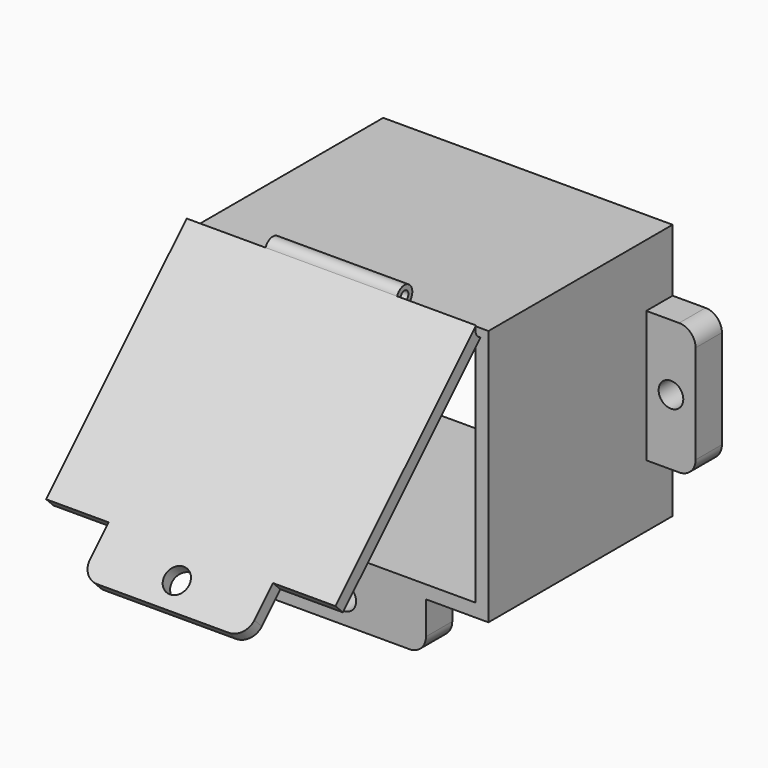
from build123d import *

# Parameters (mm, degrees)
F0_W           = 80
F0_H           = 70
F1_DEPTH       = 70
F0_W_2         = 15
F0_H_2         = 40
F0_R           = 3.75
F2_DEPTH       = 10
F3_R           = 5
F6_W           = 50
F6_H           = 15
F6_R           = 3.75
F7_DEPTH       = 10
F8_R           = 5
F9_R           = 3
F9_R_2         = 1.5
F10_DEPTH      = 20
F13_END_RADIUS = 3
F12_W          = 88
F12_H          = 4
F13_REACH      = 196.483987292
F14_R          = 3.75
F15_DEPTH      = 4
F16_R          = 5


with BuildPart() as f1:
    # F0 (on Front) → F1 (new body)
    with BuildSketch(Plane.XZ):
        Polygon((44, 39), (-44, 39), (-44, -39), (44, -39), (44, -20), (44, 20), align=None)
        Rectangle(F0_W, F0_H, mode=Mode.SUBTRACT)
    extrude(amount=F1_DEPTH)

    # F0 (on Front) → F2 (join)
    with BuildSketch(Plane.XZ):
        with Locations((51.5, 0)):
            Rectangle(F0_W_2, F0_H_2)
        with Locations((51.5, 0)):
            Circle(F0_R, mode=Mode.SUBTRACT)
    extrude(amount=F2_DEPTH)

    # F3
    f3_edges = [f1.edges().sort_by_distance(p)[0] for p in [
        (59, -5, 20),
        (59, -5, -20),
    ]]
    fillet(f3_edges, radius=F3_R)

    # F4: F1 across plane


with BuildPart() as f1_1:
    add(f1.part)
    add(f1.part.mirror(Plane.YZ))

    # F6 (on face) → F7 (join)
    with BuildSketch(Plane.XZ.offset(70)):
        with Locations((0, -46.5)):
            Rectangle(F6_W, F6_H)
        with Locations((0, -46.5)):
            Circle(F6_R, mode=Mode.SUBTRACT)
    extrude(amount=-F7_DEPTH)

    # F8
    f8_edges = [f1_1.edges().sort_by_distance(p)[0] for p in [
        (25, -65, -54),
        (-25, -65, -54),
    ]]
    fillet(f8_edges, radius=F8_R)


with BuildPart() as f10:
    # F9 (on Right) → F10 (new body, symmetric)
    with BuildSketch(Plane.YZ):
        with Locations((-71.9384711885, 41.2896133847)):
            Circle(F9_R)
        with Locations((-71.9384711885, 41.2896133847)):
            Circle(F9_R_2, mode=Mode.SUBTRACT)
    extrude(amount=F10_DEPTH, both=True)

    f13_end = (Plane(origin=(0, -71.9384711885, 41.2896133847), x_dir=(0, 0, 1), z_dir=(1, 0, 0)) * Cylinder(F13_END_RADIUS, 734.7317676539, mode=Mode.PRIVATE)).faces().sort_by_distance((0, -74.9384711885, 41.2896133847))[0]
    # F12 (on face) → F13 (join, up to the whole of a round face its end follows)
    with BuildSketch(Plane(origin=(0, -54.5, -54.5), x_dir=(-1, 0, 0), z_dir=(0, 0.7071067812, 0.7071067812))):
        with Locations((0, 80.8292925358)):
            Rectangle(F12_W, F12_H)
    f13_long = extrude(amount=F13_REACH, mode=Mode.PRIVATE)
    add(split(f13_long, bisect_by=f13_end, keep=Keep.ALL, mode=Mode.PRIVATE).solids().sort_by_distance((0, -111.6549408706, 2.6549408706))[0])

    # F14 (on face) → F15 (join)
    with BuildSketch(Plane(origin=(0, -58.5691544329, 58.5691544329), x_dir=(1, 0, 0), z_dir=(0, -0.7071067812, 0.7071067812))):
        Polygon((44, -77.0746391493), (-44, -77.0746391493), (-44, -98.4056391493), (-25, -98.4056391493), (-25, -113.4056391493), (25, -113.4056391493), (25, -98.4056391493), (44, -98.4056391493), align=None)
        with Locations((0, -105.9056391493)):
            Circle(F14_R, mode=Mode.SUBTRACT)
    extrude(amount=-F15_DEPTH)

    # F16
    f16_edges = [f10.edges().sort_by_distance(p)[0] for p in [
        (25, -137.344837, -23.034956),
        (-25, -137.344837, -23.034956),
    ]]
    fillet(f16_edges, radius=F16_R)


with BuildPart() as f10_1:
    # F17: moved
    add(f10.part)


solid = Compound([f1_1.part, f10_1.part])
